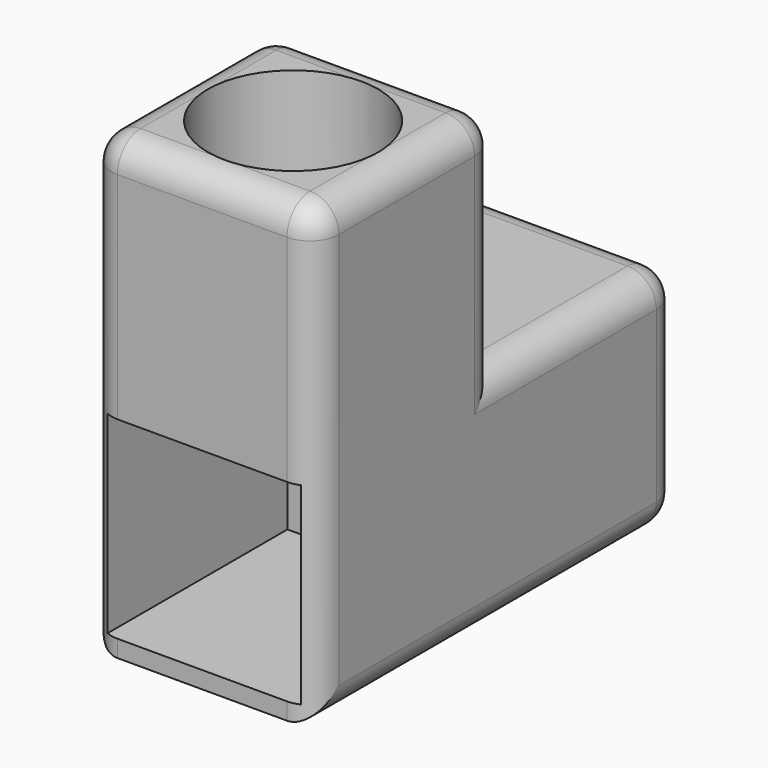
from build123d import *

# Parameters (mm, degrees)
F0_W          = 40
F0_H          = 80
F1_DEPTH      = 40
F2_W          = 40
F2_H          = 40
F3_DEPTH      = 40
F4_W          = 34
F4_H          = 34
F5_DEPTH      = 40
F6_R          = 15
F7_DEPTH      = 43
F8_R          = 10
F9_DEPTH      = 80.001
F10_T1_DEPTH  = 87.62
F10_T3_DEPTH  = 29.84
F10_T5_DEPTH  = 34.92
F10_T7_DEPTH  = 34.92
F10_T9_DEPTH  = 29.84
F10_T11_DEPTH = 87.62
F10_T13_DEPTH = 29.84
F10_S17_W     = 5.08
F10_S17_H     = 5.08
F10_T18_DEPTH = 5.08
F10_S23_W     = 5.08
F10_S23_H     = 5.08
F10_T24_DEPTH = 5.08
F10_S29_W     = 5.08
F10_S29_H     = 5.08
F10_T30_DEPTH = 5.08
F10_S35_W     = 5.08
F10_S35_H     = 5.08
F10_T36_DEPTH = 5.08
F10_S41_W     = 5.08
F10_S41_H     = 5.08
F10_T42_DEPTH = 5.08
F10_S47_W     = 5.08
F10_S47_H     = 5.08
F10_T48_DEPTH = 5.08
F10_S53_W     = 5.08
F10_S53_H     = 5.08
F10_T54_DEPTH = 5.08
F10_S59_W     = 5.08
F10_S59_H     = 5.08
F10_T60_DEPTH = 5.08
F10_T69_DEPTH = 47.62
F10_T73_DEPTH = 47.62
F10_T80_DEPTH = 47.62
F10_T84_DEPTH = 47.62


# Not quite as in the source:
# - a fillet or chamfer that OpenCascade refuses, or shapes differently, is made with other operations: its cross-section is extruded or revolved along the edge and cut away or added


with BuildPart() as f1:
    # F0 (on Top) → F1 (new body)
    with BuildSketch(Plane.XY):
        with Locations((0.2714497969, 6.1442126253)):
            Rectangle(F0_W, F0_H)
    extrude(amount=F1_DEPTH)

    # F2 (on face) → F3 (join)
    with BuildSketch(Plane.XY.offset(40)):
        with Locations((0.2714497969, -13.8557873747)):
            Rectangle(F2_W, F2_H)
    extrude(amount=F3_DEPTH)

    # F4 (on face) → F5 (cut)
    with BuildSketch(Plane.XZ.offset(33.8557873747)):
        with Locations((0.2714497969, 20)):
            Rectangle(F4_W, F4_H)
    extrude(amount=-F5_DEPTH, mode=Mode.SUBTRACT)

    # F6 (on face) → F7 (cut, through all)
    with BuildSketch(Plane.XY.offset(80)):
        with Locations((0.2714497969, -13.8557873747)):
            Circle(F6_R)
    extrude(amount=-F7_DEPTH, mode=Mode.SUBTRACT)

    # F8 (on face) → F9 (cut, through all)
    with BuildSketch(Plane(origin=(0, 46.1442126253, 0), x_dir=(-1, 0, 0), z_dir=(0, 1, 0))):
        with Locations((0, 20)):
            Circle(F8_R)
    extrude(amount=-F9_DEPTH, mode=Mode.SUBTRACT)

    # F10: fillet of radius 5.08 on 17 edges, made by hand

    # F10_s2 → F10_t1 (cut)
    with BuildSketch(Plane.XY.offset(-12.7)):
        with BuildLine():
            ThreePointArc((20.2714497969, -28.7757873747), (18.7835522453, -32.3678898231), (15.1914497969, -33.8557873747))
            Line((15.1914497969, -33.8557873747), (20.2714497969, -33.8557873747))
            Line((20.2714497969, -33.8557873747), (20.2714497969, -28.7757873747))
        make_face()
        with BuildLine():
            ThreePointArc((-19.7285502031, -28.7757873747), (-18.2406526516, -32.3678898231), (-14.6485502031, -33.8557873747))
            Line((-14.6485502031, -33.8557873747), (-19.7285502031, -33.8557873747))
            Line((-19.7285502031, -33.8557873747), (-19.7285502031, -28.7757873747))
        make_face()
    extrude(amount=F10_T1_DEPTH, mode=Mode.SUBTRACT)

    # F10_s4 → F10_t3 (cut)
    with BuildSketch(Plane.XZ.offset(-1.0642126253)):
        with BuildLine():
            ThreePointArc((20.2714497969, 74.92), (18.7835522453, 78.5121024484), (15.1914497969, 80))
            Line((15.1914497969, 80), (20.2714497969, 80))
            Line((20.2714497969, 80), (20.2714497969, 74.92))
        make_face()
        with BuildLine():
            ThreePointArc((-19.7285502031, 74.92), (-18.2406526516, 78.5121024484), (-14.6485502031, 80))
            Line((-14.6485502031, 80), (-19.7285502031, 80))
            Line((-19.7285502031, 80), (-19.7285502031, 74.92))
        make_face()
    extrude(amount=F10_T3_DEPTH, mode=Mode.SUBTRACT)

    # F10_s6 → F10_t5 (cut)
    with BuildSketch(Plane.XY.offset(40)):
        with BuildLine():
            ThreePointArc((20.2714497969, 1.0642126253), (18.7835522453, 4.6563150738), (15.1914497969, 6.1442126253))
            Line((15.1914497969, 6.1442126253), (20.2714497969, 6.1442126253))
            Line((20.2714497969, 6.1442126253), (20.2714497969, 1.0642126253))
        make_face()
        with BuildLine():
            ThreePointArc((-19.7285502031, 1.0642126253), (-18.2406526516, 4.6563150738), (-14.6485502031, 6.1442126253))
            Line((-14.6485502031, 6.1442126253), (-19.7285502031, 6.1442126253))
            Line((-19.7285502031, 6.1442126253), (-19.7285502031, 1.0642126253))
        make_face()
    extrude(amount=F10_T5_DEPTH, mode=Mode.SUBTRACT)

    # F10_s8 → F10_t7 (cut)
    with BuildSketch(Plane.XZ.offset(-41.0642126253)):
        with BuildLine():
            ThreePointArc((20.2714497969, 34.92), (18.7835522453, 38.5121024484), (15.1914497969, 40))
            Line((15.1914497969, 40), (20.2714497969, 40))
            Line((20.2714497969, 40), (20.2714497969, 34.92))
        make_face()
        with BuildLine():
            ThreePointArc((-14.6485502031, 40), (-18.2406526516, 38.5121024484), (-19.7285502031, 34.92))
            Line((-19.7285502031, 34.92), (-19.7285502031, 40))
            Line((-19.7285502031, 40), (-14.6485502031, 40))
        make_face()
    extrude(amount=F10_T7_DEPTH, mode=Mode.SUBTRACT)

    # F10_s10 → F10_t9 (cut)
    with BuildSketch(Plane.XY.offset(5.08)):
        with BuildLine():
            ThreePointArc((15.1914497969, 46.1442126253), (18.7835522453, 44.6563150738), (20.2714497969, 41.0642126253))
            Line((20.2714497969, 41.0642126253), (20.2714497969, 46.1442126253))
            Line((20.2714497969, 46.1442126253), (15.1914497969, 46.1442126253))
        make_face()
        with BuildLine():
            ThreePointArc((-14.6485502031, 46.1442126253), (-18.2406526516, 44.6563150738), (-19.7285502031, 41.0642126253))
            Line((-19.7285502031, 41.0642126253), (-19.7285502031, 46.1442126253))
            Line((-19.7285502031, 46.1442126253), (-14.6485502031, 46.1442126253))
        make_face()
    extrude(amount=F10_T9_DEPTH, mode=Mode.SUBTRACT)

    # F10_s12 → F10_t11 (cut)
    with BuildSketch(Plane.XZ.offset(-41.0642126253)):
        with BuildLine():
            ThreePointArc((20.2714497969, 5.08), (18.7835522453, 1.4878975516), (15.1914497969, 0))
            Line((15.1914497969, 0), (20.2714497969, 0))
            Line((20.2714497969, 0), (20.2714497969, 5.08))
        make_face()
        with BuildLine():
            ThreePointArc((-14.6485502031, 0), (-18.2406526516, 1.4878975516), (-19.7285502031, 5.08))
            Line((-19.7285502031, 5.08), (-19.7285502031, 0))
            Line((-19.7285502031, 0), (-14.6485502031, 0))
        make_face()
    extrude(amount=F10_T11_DEPTH, mode=Mode.SUBTRACT)

    # F10_s14 → F10_t13 (cut)
    with BuildSketch(Plane.YZ.offset(-14.6485502031)):
        with BuildLine():
            ThreePointArc((46.1442126253, 5.08), (44.6563150738, 1.4878975516), (41.0642126253, 0))
            Line((41.0642126253, 0), (46.1442126253, 0))
            Line((46.1442126253, 0), (46.1442126253, 5.08))
        make_face()
        with BuildLine():
            ThreePointArc((46.1442126253, 34.92), (44.6563150738, 38.5121024484), (41.0642126253, 40))
            Line((41.0642126253, 40), (46.1442126253, 40))
            Line((46.1442126253, 40), (46.1442126253, 34.92))
        make_face()
        with BuildLine():
            ThreePointArc((-33.8557873747, 74.92), (-32.3678898231, 78.5121024484), (-28.7757873747, 80))
            Line((-28.7757873747, 80), (-33.8557873747, 80))
            Line((-33.8557873747, 80), (-33.8557873747, 74.92))
        make_face()
        with BuildLine():
            ThreePointArc((1.0642126253, 80), (4.6563150738, 78.5121024484), (6.1442126253, 74.92))
            Line((6.1442126253, 74.92), (6.1442126253, 80))
            Line((6.1442126253, 80), (1.0642126253, 80))
        make_face()
    extrude(amount=F10_T13_DEPTH, mode=Mode.SUBTRACT)


with BuildPart() as f10_tool16:
    # F10_s17 → F10_t18 (new body)
    with BuildSketch(Plane.YZ.offset(15.1914497969)):
        with Locations((-31.3157873747, 77.46)):
            Rectangle(F10_S17_W, F10_S17_H)
    extrude(amount=F10_T18_DEPTH)

    # F10_s19 → F10_t20 (revolve, cut)
    with BuildSketch(Plane(origin=(15.1914497969, -28.7757873747, 74.92), x_dir=(0, 0.7071067812, -0.7071067812), z_dir=(0, -0.7071067812, -0.7071067812))):
        with BuildLine():
            ThreePointArc((0, -5.08), (5.08, 0), (0, 5.08))
            Line((0, 5.08), (0, -5.08))
        make_face()
    revolve(axis=Axis((15.1914497969, -28.7757873747, 74.92), (1, 0, 0)), mode=Mode.SUBTRACT)


with BuildPart() as f1_1:
    add(f1.part)

    # F10_t15: cut F10_tool16
    add(f10_tool16.part, mode=Mode.SUBTRACT)


with BuildPart() as f10_tool22:
    # F10_s23 → F10_t24 (new body)
    with BuildSketch(Plane.XZ.offset(-1.0642126253)):
        with Locations((17.7314497969, 77.46)):
            Rectangle(F10_S23_W, F10_S23_H)
    extrude(amount=-F10_T24_DEPTH)

    # F10_s25 → F10_t26 (revolve, cut)
    with BuildSketch(Plane(origin=(15.1914497969, 1.0642126253, 74.92), x_dir=(-0.7071067812, 0, -0.7071067812), z_dir=(0.7071067812, 0, -0.7071067812))):
        with BuildLine():
            ThreePointArc((0, -5.08), (5.08, 0), (0, 5.08))
            Line((0, 5.08), (0, -5.08))
        make_face()
    revolve(axis=Axis((15.1914497969, 1.0642126253, 74.92), (0, 1, 0)), mode=Mode.SUBTRACT)


with BuildPart() as f1_2:
    add(f1_1.part)

    # F10_t21: cut F10_tool22
    add(f10_tool22.part, mode=Mode.SUBTRACT)


with BuildPart() as f10_tool28:
    # F10_s29 → F10_t30 (new body)
    with BuildSketch(Plane.XZ.offset(-41.0642126253)):
        with Locations((17.7314497969, 37.46)):
            Rectangle(F10_S29_W, F10_S29_H)
    extrude(amount=-F10_T30_DEPTH)

    # F10_s31 → F10_t32 (revolve, cut)
    with BuildSketch(Plane(origin=(15.1914497969, 41.0642126253, 34.92), x_dir=(-0.7071067812, 0, -0.7071067812), z_dir=(0.7071067812, 0, -0.7071067812))):
        with BuildLine():
            ThreePointArc((0, -5.08), (5.08, 0), (0, 5.08))
            Line((0, 5.08), (0, -5.08))
        make_face()
    revolve(axis=Axis((15.1914497969, 41.0642126253, 34.92), (0, 1, 0)), mode=Mode.SUBTRACT)


with BuildPart() as f1_3:
    add(f1_2.part)

    # F10_t27: cut F10_tool28
    add(f10_tool28.part, mode=Mode.SUBTRACT)


with BuildPart() as f10_tool34:
    # F10_s35 → F10_t36 (new body)
    with BuildSketch(Plane.XZ.offset(-41.0642126253)):
        with Locations((17.7314497969, 2.54)):
            Rectangle(F10_S35_W, F10_S35_H)
    extrude(amount=-F10_T36_DEPTH)

    # F10_s37 → F10_t38 (revolve, cut)
    with BuildSketch(Plane(origin=(15.1914497969, 41.0642126253, 5.08), x_dir=(-0.7071067812, 0, 0.7071067812), z_dir=(-0.7071067812, 0, -0.7071067812))):
        with BuildLine():
            ThreePointArc((0, -5.08), (5.08, 0), (0, 5.08))
            Line((0, 5.08), (0, -5.08))
        make_face()
    revolve(axis=Axis((15.1914497969, 41.0642126253, 5.08), (0, 1, 0)), mode=Mode.SUBTRACT)


with BuildPart() as f1_4:
    add(f1_3.part)

    # F10_t33: cut F10_tool34
    add(f10_tool34.part, mode=Mode.SUBTRACT)


with BuildPart() as f10_tool40:
    # F10_s41 → F10_t42 (new body)
    with BuildSketch(Plane.XZ.offset(-41.0642126253)):
        with Locations((-17.1885502031, 2.54)):
            Rectangle(F10_S41_W, F10_S41_H)
    extrude(amount=-F10_T42_DEPTH)

    # F10_s43 → F10_t44 (revolve, cut)
    with BuildSketch(Plane(origin=(-14.6485502031, 41.0642126253, 5.08), x_dir=(0.7071067812, 0, 0.7071067812), z_dir=(-0.7071067812, 0, 0.7071067812))):
        with BuildLine():
            ThreePointArc((0, -5.08), (5.08, 0), (0, 5.08))
            Line((0, 5.08), (0, -5.08))
        make_face()
    revolve(axis=Axis((-14.6485502031, 41.0642126253, 5.08), (0, 1, 0)), mode=Mode.SUBTRACT)


with BuildPart() as f1_5:
    add(f1_4.part)

    # F10_t39: cut F10_tool40
    add(f10_tool40.part, mode=Mode.SUBTRACT)


with BuildPart() as f10_tool46:
    # F10_s47 → F10_t48 (new body)
    with BuildSketch(Plane.XZ.offset(-41.0642126253)):
        with Locations((-17.1885502031, 37.46)):
            Rectangle(F10_S47_W, F10_S47_H)
    extrude(amount=-F10_T48_DEPTH)

    # F10_s49 → F10_t50 (revolve, cut)
    with BuildSketch(Plane(origin=(-14.6485502031, 41.0642126253, 34.92), x_dir=(0.7071067812, 0, -0.7071067812), z_dir=(0.7071067812, 0, 0.7071067812))):
        with BuildLine():
            ThreePointArc((0, -5.08), (5.08, 0), (0, 5.08))
            Line((0, 5.08), (0, -5.08))
        make_face()
    revolve(axis=Axis((-14.6485502031, 41.0642126253, 34.92), (0, 1, 0)), mode=Mode.SUBTRACT)


with BuildPart() as f1_6:
    add(f1_5.part)

    # F10_t45: cut F10_tool46
    add(f10_tool46.part, mode=Mode.SUBTRACT)


with BuildPart() as f10_tool52:
    # F10_s53 → F10_t54 (new body)
    with BuildSketch(Plane.XZ.offset(-1.0642126253)):
        with Locations((-17.1885502031, 77.46)):
            Rectangle(F10_S53_W, F10_S53_H)
    extrude(amount=-F10_T54_DEPTH)

    # F10_s55 → F10_t56 (revolve, cut)
    with BuildSketch(Plane(origin=(-14.6485502031, 1.0642126253, 74.92), x_dir=(0.7071067812, 0, -0.7071067812), z_dir=(0.7071067812, 0, 0.7071067812))):
        with BuildLine():
            ThreePointArc((0, -5.08), (5.08, 0), (0, 5.08))
            Line((0, 5.08), (0, -5.08))
        make_face()
    revolve(axis=Axis((-14.6485502031, 1.0642126253, 74.92), (0, 1, 0)), mode=Mode.SUBTRACT)


with BuildPart() as f1_7:
    add(f1_6.part)

    # F10_t51: cut F10_tool52
    add(f10_tool52.part, mode=Mode.SUBTRACT)


with BuildPart() as f10_tool58:
    # F10_s59 → F10_t60 (new body)
    with BuildSketch(Plane.YZ.offset(-14.6485502031)):
        with Locations((-31.3157873747, 77.46)):
            Rectangle(F10_S59_W, F10_S59_H)
    extrude(amount=-F10_T60_DEPTH)

    # F10_s61 → F10_t62 (revolve, cut)
    with BuildSketch(Plane(origin=(-14.6485502031, -28.7757873747, 74.92), x_dir=(0, 0.7071067812, -0.7071067812), z_dir=(0, 0.7071067812, 0.7071067812))):
        with BuildLine():
            ThreePointArc((0, -5.08), (5.08, 0), (0, 5.08))
            Line((0, 5.08), (0, -5.08))
        make_face()
    revolve(axis=Axis((-14.6485502031, -28.7757873747, 74.92), (-1, 0, 0)), mode=Mode.SUBTRACT)


with BuildPart() as f1_8:
    add(f1_7.part)

    # F10_t57: cut F10_tool58
    add(f10_tool58.part, mode=Mode.SUBTRACT)

    # F10_s63 → F10_t64 (revolve, cut)
    with BuildSketch(Plane.XY.offset(20)):
        with BuildLine():
            ThreePointArc((-15.08, 46.1442126253), (-11.4878975516, 44.6563150738), (-10, 41.0642126253))
            Line((-10, 41.0642126253), (-10, 46.1442126253))
            Line((-10, 46.1442126253), (-15.08, 46.1442126253))
        make_face()
    revolve(axis=Axis((0, 46.1442126253, 20), (0, 1, 0)), mode=Mode.SUBTRACT)


with BuildPart() as f10_tool67:
    # F10_s68 → F10_t69 (new body)
    with BuildSketch(Plane.XY.offset(27.3)):
        with BuildLine():
            ThreePointArc((20.2714497969, 1.0642126253), (18.7835522453, 4.6563150738), (15.1914497969, 6.1442126253))
            Line((15.1914497969, 6.1442126253), (20.2714497969, 6.1442126253))
            Line((20.2714497969, 6.1442126253), (20.2714497969, 1.0642126253))
        make_face()
    extrude(amount=F10_T69_DEPTH)

    split(bisect_by=Plane.XY.offset(40), keep=Keep.BOTTOM)


with BuildPart() as f10_tool71:
    # F10_s72 → F10_t73 (new body)
    with BuildSketch(Plane.XZ.offset(6.5557873747)):
        with BuildLine():
            ThreePointArc((20.2714497969, 34.92), (18.7835522453, 38.5121024484), (15.1914497969, 40))
            Line((15.1914497969, 40), (20.2714497969, 40))
            Line((20.2714497969, 40), (20.2714497969, 34.92))
        make_face()
    extrude(amount=-F10_T73_DEPTH)

    split(bisect_by=Plane.XZ.offset(-6.1442126253), keep=Keep.TOP)


with BuildPart() as f10_tool67_1:
    add(f10_tool67.part)

    # F10_t75: intersect F10_tool71
    add(f10_tool71.part, mode=Mode.INTERSECT)


with BuildPart() as f1_9:
    add(f1_8.part)

    # F10_t65: cut F10_tool67
    add(f10_tool67_1.part, mode=Mode.SUBTRACT)


with BuildPart() as f10_tool78:
    # F10_s79 → F10_t80 (new body)
    with BuildSketch(Plane.XZ.offset(-41.0642126253)):
        with BuildLine():
            ThreePointArc((-14.6485502031, 40), (-18.2406526516, 38.5121024484), (-19.7285502031, 34.92))
            Line((-19.7285502031, 34.92), (-19.7285502031, 40))
            Line((-19.7285502031, 40), (-14.6485502031, 40))
        make_face()
    extrude(amount=F10_T80_DEPTH)

    split(bisect_by=Plane.XZ.offset(-6.1442126253), keep=Keep.TOP)


with BuildPart() as f10_tool82:
    # F10_s83 → F10_t84 (new body)
    with BuildSketch(Plane.XY.offset(27.3)):
        with BuildLine():
            ThreePointArc((-19.7285502031, 1.0642126253), (-18.2406526516, 4.6563150738), (-14.6485502031, 6.1442126253))
            Line((-14.6485502031, 6.1442126253), (-19.7285502031, 6.1442126253))
            Line((-19.7285502031, 6.1442126253), (-19.7285502031, 1.0642126253))
        make_face()
    extrude(amount=F10_T84_DEPTH)

    split(bisect_by=Plane.XY.offset(40), keep=Keep.BOTTOM)


with BuildPart() as f10_tool78_1:
    add(f10_tool78.part)

    # F10_t86: intersect F10_tool82
    add(f10_tool82.part, mode=Mode.INTERSECT)


with BuildPart() as f1_10:
    add(f1_9.part)

    # F10_t76: cut F10_tool78
    add(f10_tool78_1.part, mode=Mode.SUBTRACT)


solid = f1_10.part
